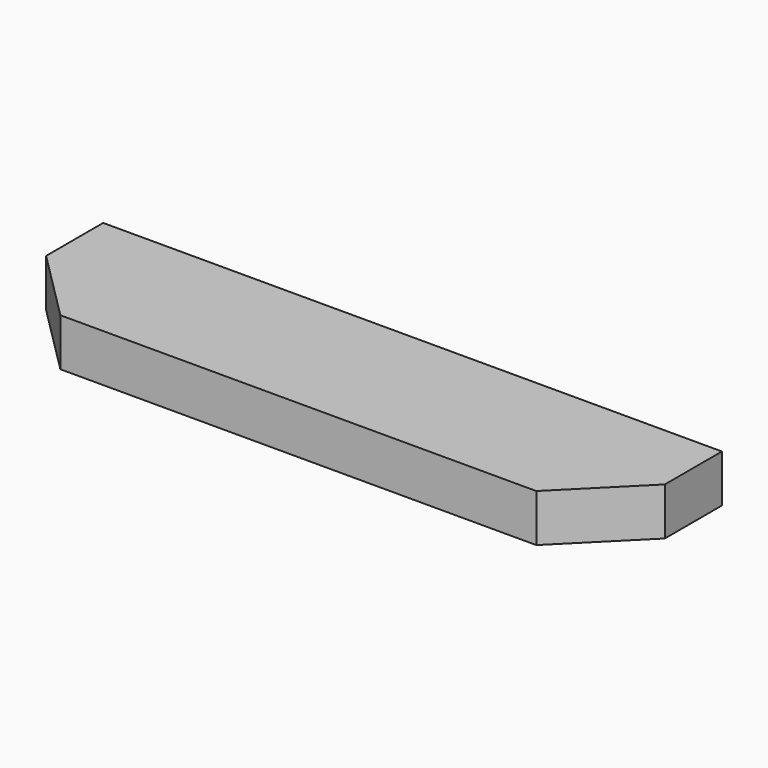
from build123d import *

# Parameters (mm, degrees)
F0_W     = 150
F0_H     = 50
F1_DEPTH = 325
F3_DEPTH = 50.001


# Not quite as in the source:
# - a pattern or mirror of a feature is missing from the dataset's text; its kind, count and spacing are read off the source's solid


with BuildPart() as f1:
    # F0 (on Right) → F1 (new body, symmetric)
    with BuildSketch(Plane.YZ):
        Rectangle(F0_W, F0_H)
    extrude(amount=F1_DEPTH, both=True)

    # F2 (on face) → F3 (cut, through all)
    with BuildSketch(Plane.XY.offset(25)):
        Polygon((-250, -75), (-325, 0), (-325, -75), align=None)
    f3 = extrude(amount=-F3_DEPTH, mode=Mode.SUBTRACT)

    # F3_copies: F3 across plane
    add(f3.mirror(Plane(origin=(0, 0, 0), x_dir=(0, 0, 1), z_dir=(1, 0, 0))), mode=Mode.SUBTRACT)


solid = f1.part
